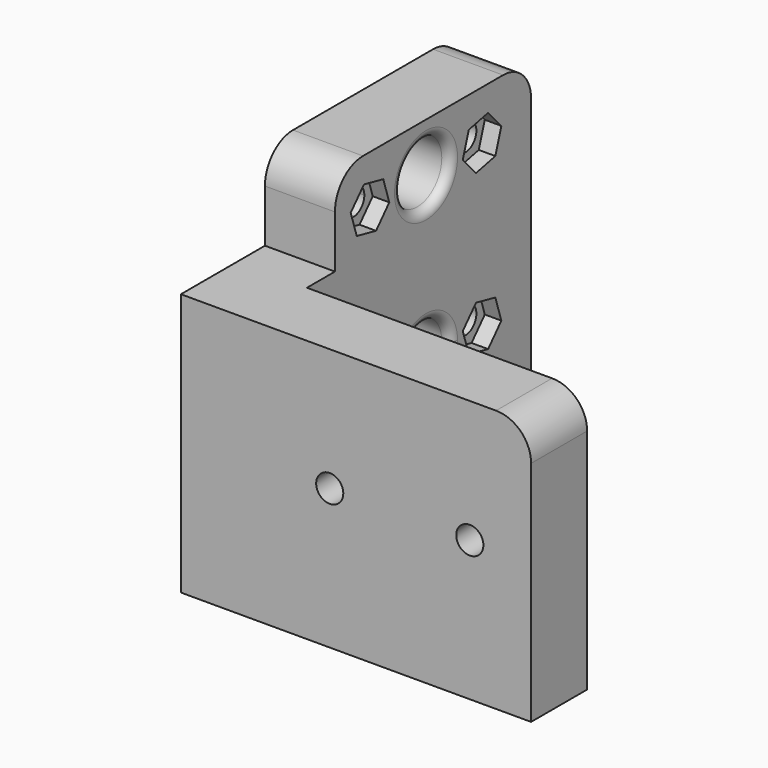
from build123d import *

# Parameters (mm, degrees)
F0_R      = 1.9722998741
F0_R_2    = 4.445
F1_DEPTH  = 10.16
F2_R      = 1.9722998741
F3_DEPTH  = 2.4
F4_R      = 5.08
F5_W      = 50.8
F5_H      = 38.1
F5_R      = 1.9685
F6_DEPTH  = 10.16
F7_R      = 5.08
F8_R      = 1.9685
F9_DEPTH  = 2.4
F11_DEPTH = 10.16
F12_R     = 1.27


# Not quite as in the source:
# - a feature names something its author has since deleted; it is built from what else it names


with BuildPart() as f1:
    # F0 (on Right) → F1 (new body)
    with BuildSketch(Plane.YZ):
        Polygon((15.24, 38.1), (0, 38.1), (0, 0), (31.75, 0), (50.8, 0), (50.8, 50.8), (31.75, 50.8), (21.59, 50.8), (15.24, 50.8), align=None)
        with Locations((21.59, 20.32)):
            Circle(F0_R, mode=Mode.SUBTRACT)
        with BuildLine():
            ThreePointArc((36.195, 20.32), (34.8930896424, 17.1769103576), (31.75, 15.875))
            ThreePointArc((31.75, 15.875), (28.6069103576, 23.4630896424), (36.195, 20.32))
        make_face(mode=Mode.SUBTRACT)
        with Locations((41.91, 20.32)):
            Circle(F0_R, mode=Mode.SUBTRACT)
        with BuildLine():
            ThreePointArc((23.5622998741, 43.688), (20.1953733845, 42.2933733845), (21.59, 45.6602998741))
            ThreePointArc((21.59, 45.6602998741), (22.9846266155, 45.0826266155), (23.5622998741, 43.688))
        make_face(mode=Mode.SUBTRACT)
        with Locations((31.75, 43.688)):
            Circle(F0_R_2, mode=Mode.SUBTRACT)
        with Locations((41.91, 43.688)):
            Circle(F0_R, mode=Mode.SUBTRACT)
    extrude(amount=F1_DEPTH)

    # F2 (on face) → F3 (cut)
    with BuildSketch(Plane.YZ.offset(10.16)):
        Polygon((20.4920916615, 47.0950413284), (18.0904614886, 44.440704152), (19.1883698271, 41.0336628236), (22.6879083385, 40.2809586716), (25.0895385114, 42.935295848), (23.9916301729, 46.3423371764), align=None)
        with Locations((21.59, 43.688)):
            Circle(F2_R, mode=Mode.SUBTRACT)
        Polygon((40.8120916615, 40.2809586716), (44.3116301729, 41.0336628236), (45.4095385114, 44.440704152), (43.0079083385, 47.0950413284), (39.5083698271, 46.3423371764), (38.4104614886, 42.935295848), align=None)
        with Locations((41.91, 43.688)):
            Circle(F2_R, mode=Mode.SUBTRACT)
        Polygon((44.3116301729, 22.9743371764), (40.8120916615, 23.7270413284), (38.4104614886, 21.072704152), (39.5083698271, 17.6656628236), (43.0079083385, 16.9129586716), (45.4095385114, 19.567295848), align=None)
        with Locations((41.91, 20.32)):
            Circle(F2_R, mode=Mode.SUBTRACT)
        Polygon((22.6879083385, 23.7270413284), (19.1883698271, 22.9743371764), (18.0904614886, 19.567295848), (20.4920916615, 16.9129586716), (23.9916301729, 17.6656628236), (25.0895385114, 21.072704152), align=None)
        with Locations((21.59, 20.32)):
            Circle(F2_R, mode=Mode.SUBTRACT)
    extrude(amount=-F3_DEPTH, mode=Mode.SUBTRACT)

    # F4
    f4_edges = [f1.edges().sort_by_distance(p)[0] for p in [
        (5.08, 50.8, 50.8),
        (5.08, 15.24, 50.8),
    ]]
    fillet(f4_edges, radius=F4_R)

    # F5 (on Front) → F6 (join)
    with BuildSketch(Plane.XZ):
        with Locations((25.4, 19.05)):
            Rectangle(F5_W, F5_H)
        with Locations((21.59, 20.32)):
            Circle(F5_R, mode=Mode.SUBTRACT)
        with Locations((41.91, 20.32)):
            Circle(F5_R, mode=Mode.SUBTRACT)
    extrude(amount=-F6_DEPTH)

    # F7
    f7_edges = [f1.edges().sort_by_distance(p)[0] for p in [
        (50.8, 5.08, 38.1),
    ]]
    fillet(f7_edges, radius=F7_R)

    # F8 (on face) → F9 (cut)
    with BuildSketch(Plane(origin=(0, 10.16, 0), x_dir=(-1, 0, 0), z_dir=(0, 1, 0))):
        Polygon((-41.2323596559, 23.8334340491), (-44.613902969, 22.6635707772), (-45.2915433131, 19.1501367281), (-42.5876403441, 16.8065659509), (-39.206097031, 17.9764292228), (-38.5284566869, 21.4898632719), align=None)
        with Locations((-41.91, 20.32)):
            Circle(F8_R, mode=Mode.SUBTRACT)
        Polygon((-24.293902969, 17.9764292228), (-20.9123596559, 16.8065659509), (-18.2084566869, 19.1501367281), (-18.886097031, 22.6635707772), (-22.2676403441, 23.8334340491), (-24.9715433131, 21.4898632719), align=None)
        with Locations((-21.59, 20.32)):
            Circle(F8_R, mode=Mode.SUBTRACT)
    extrude(amount=-F9_DEPTH, mode=Mode.SUBTRACT)

    # F10 (on face) → F11 (join)
    with BuildSketch(Plane(origin=(0, 0, 0), x_dir=(1, 0, 0), z_dir=(0, 0, -1))):
        Polygon((10.16, -10.16), (10.16, -50.8), (50.8, -10.16), align=None)
    extrude(amount=-F11_DEPTH)

    # F12
    f12_edges = [f1.edges().sort_by_distance(p)[0] for p in [
        (10.16, 27.305, 20.32),
        (10.16, 27.305, 43.688),
    ]]
    fillet(f12_edges, radius=F12_R)


solid = f1.part
